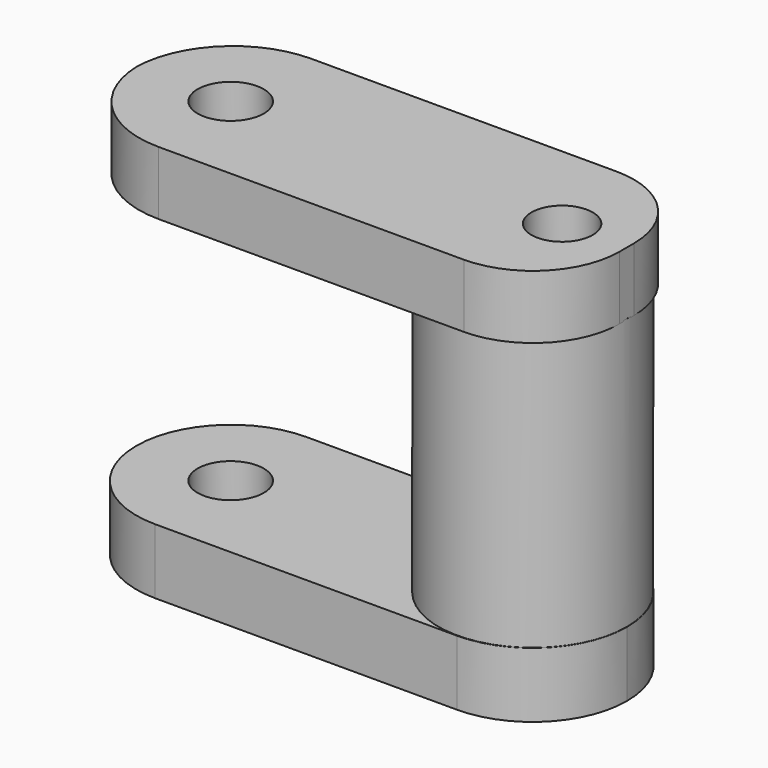
from build123d import *

# Parameters (mm, degrees)
F0_W         = 153.0012339354
F0_H         = 58.951575309
F1_DEPTH     = 20.32
F2_R         = 29.4340917525
F3_R         = 29.3662882484
F3_R_2       = 9.1215869303
F4_DEPTH     = 84.582
F5_DEPTH     = 84.583
F6_R         = 12.0800155098
F7_DEPTH     = 84.583
F9_W         = 152.801066637
F9_H         = 59.5563165843
F10_DEPTH    = 19.812
F11_R        = 10.3122867818
F12_DEPTH    = 124.461
F13_T1_DEPTH = 173.1145612107
F14_R        = 26.9812507731
F15_R        = 9.5592417263
F16_DEPTH    = 124.461


# Not quite as in the source:
# - a fillet or chamfer that OpenCascade refuses, or shapes differently, is made with other operations: its cross-section is extruded or revolved along the edge and cut away or added


with BuildPart() as f1:
    # F0 (on Top) → F1 (new body)
    with BuildSketch(Plane.XY):
        Rectangle(F0_W, F0_H)
    extrude(amount=F1_DEPTH)

    # F2
    f2_edges = [f1.edges().sort_by_distance(p)[0] for p in [
        (-76.500617, -29.475788, 10.16),
        (-76.500617, 29.475788, 10.16),
        (76.500617, -29.475788, 10.16),
        (76.500617, 29.475788, 10.16),
    ]]
    fillet(f2_edges, radius=F2_R)

    # F3 (on face) → F4 (join)
    with BuildSketch(Plane.XY.offset(20.32)):
        with Locations((47.0665252152, 0.0416959021)):
            Circle(F3_R)
        with Locations((47.0665252152, 0.0416959021)):
            Circle(F3_R_2, mode=Mode.SUBTRACT)
    extrude(amount=F4_DEPTH)

    # F5 (cut, through all): a face of the model
    f5_faces = [f1.faces().sort_by_distance(p)[0] for p in [
        (47.0665252152, 0.0416959021, 20.32),
    ]]
    extrude(f5_faces, amount=F5_DEPTH, mode=Mode.SUBTRACT)

    # F6 (on face) → F7 (cut, through all)
    with BuildSketch(Plane.XY.offset(20.32)):
        with Locations((-47.0665252152, 0.0416959021)):
            Circle(F6_R)
    extrude(amount=F7_DEPTH, mode=Mode.SUBTRACT)

    # F9 (on offset) → F10 (join)
    with BuildSketch(Plane.XY.offset(104.648)):
        Rectangle(F9_W, F9_H)
    extrude(amount=F10_DEPTH)

    # F11 (on face) → F12 (cut, through all)
    with BuildSketch(Plane(origin=(0, 0, 0), x_dir=(1, 0, 0), z_dir=(0, 0, -1))):
        with Locations((-47.0665252152, 0.0416959021)):
            Circle(F11_R)
    extrude(amount=-F12_DEPTH, mode=Mode.SUBTRACT)

    # F13: fillet of radius 30.6605122421 on 2 edges, made by hand

    # F13_s2 → F13_t1 (cut)
    with BuildSketch(Plane.XY.offset(27.9967193947)):
        with BuildLine():
            ThreePointArc((-45.7400210764, -29.7781582922), (-67.4202771975, -20.7979021711), (-76.4005333185, 0.88235395))
            Line((-76.4005333185, 0.88235395), (-76.4005333185, -29.7781582922))
            Line((-76.4005333185, -29.7781582922), (-45.7400210764, -29.7781582922))
        make_face()
        with BuildLine():
            ThreePointArc((-45.7400210764, 29.7781582922), (-67.4202771975, 20.7979021711), (-76.4005333185, -0.88235395))
            Line((-76.4005333185, -0.88235395), (-76.4005333185, 29.7781582922))
            Line((-76.4005333185, 29.7781582922), (-45.7400210764, 29.7781582922))
        make_face()
    extrude(amount=F13_T1_DEPTH, mode=Mode.SUBTRACT)

    # F14
    f14_edges = [f1.edges().sort_by_distance(p)[0] for p in [
        (76.400533, -29.778158, 114.554),
        (76.400533, 29.778158, 114.554),
    ]]
    fillet(f14_edges, radius=F14_R)

    # F15 (on face) → F16 (cut, through all)
    with BuildSketch(Plane(origin=(0, 0, 0), x_dir=(1, 0, 0), z_dir=(0, 0, -1))):
        with Locations((56.2476292253, 0)):
            Circle(F15_R)
    extrude(amount=-F16_DEPTH, mode=Mode.SUBTRACT)


solid = f1.part
